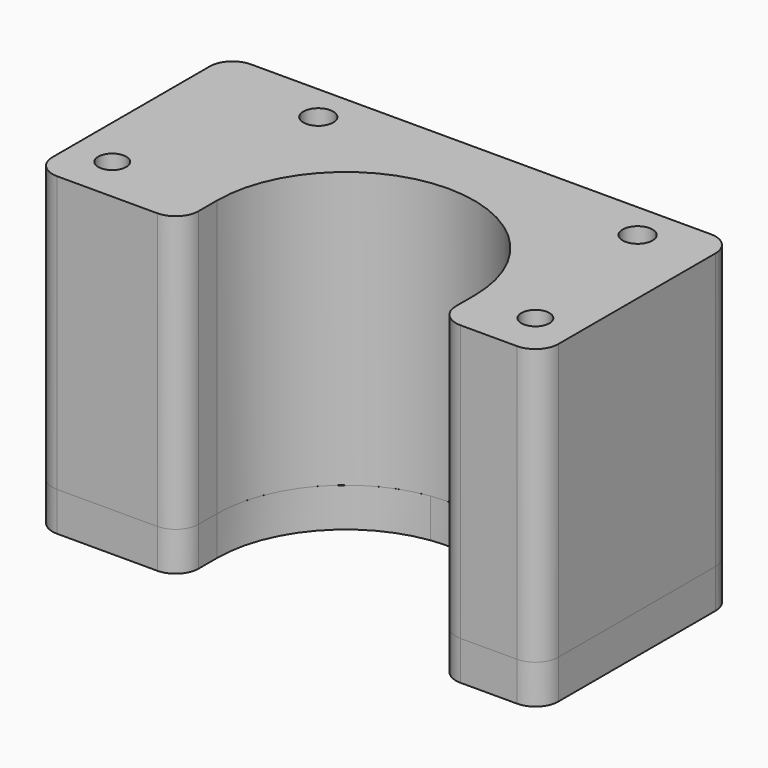
from build123d import *

# Parameters (mm, degrees)
F2_R     = 5.5
F2_R_2   = 3.25
F2_R_3   = 2.5
F2_R_4   = 3.05
F2_R_5   = 2.79
F3_DEPTH = 8.5
F4_R     = 5
F5_R     = 5.5
F5_R_2   = 3.25
F6_DEPTH = 10
F7_R     = 5.5
F7_R_2   = 3.25
F7_R_3   = 3.05
F8_DEPTH = 50


# Not quite as in the source:
# - a feature names something its author has since deleted; it is built from what else it names


with BuildPart() as f3:
    # F2 (on offset) → F3 (new body)
    with BuildSketch(Plane.XY.offset(-60)):
        with BuildLine():
            ThreePointArc((-3.739333985, 27.7491870394), (-12.178842961, 33.2301269514), (-15.455, 42.745))
            Line((-15.455, 42.745), (-59.8, 42.745))
            Line((-59.8, 42.745), (-59.8, -10))
            Line((-59.8, -10), (-28, -10))
            Line((-28, -10), (-28, 0))
            ThreePointArc((-28, 0), (-21.0796270316, 18.429577429), (-3.739333985, 27.7491870394))
        make_face()
        with Locations((-50.8, 0)):
            Circle(F2_R, mode=Mode.SUBTRACT)
        with Locations((-33.75, 34.745)):
            Circle(F2_R_2, mode=Mode.SUBTRACT)
        with BuildLine():
            Line((50.3, 42.745), (15.455, 42.745))
            ThreePointArc((15.455, 42.745), (12.178842961, 33.2301269514), (3.739333985, 27.7491870394))
            ThreePointArc((3.739333985, 27.7491870394), (21.0796270316, 18.429577429), (28, 0))
            Line((28, 0), (28, -10))
            Line((28, -10), (50.3, -10))
            Line((50.3, -10), (50.3, 42.745))
        make_face()
        with Locations((41.3, 0)):
            Circle(F2_R, mode=Mode.SUBTRACT)
        with Locations((35.75, 34.745)):
            Circle(F2_R_2, mode=Mode.SUBTRACT)
        with BuildLine():
            Line((-15.455, 42.745), (15.455, 42.745))
            ThreePointArc((15.455, 42.745), (0, 58.2), (-15.455, 42.745))
        make_face()
        with Locations((0, 52.7)):
            Circle(F2_R_3, mode=Mode.SUBTRACT)
        with BuildLine():
            ThreePointArc((3.739333985, 27.7491870394), (12.178842961, 33.2301269514), (15.455, 42.745))
            Line((15.455, 42.745), (-15.455, 42.745))
            ThreePointArc((-15.455, 42.745), (-12.178842961, 33.2301269514), (-3.739333985, 27.7491870394))
            ThreePointArc((-3.739333985, 27.7491870394), (0, 28), (3.739333985, 27.7491870394))
        make_face()
        with Locations((-50.8, 0)):
            Circle(F2_R)
        with Locations((-50.8, 0)):
            Circle(F2_R_4, mode=Mode.SUBTRACT)
        with Locations((41.3, 0)):
            Circle(F2_R)
        with Locations((41.3, 0)):
            Circle(F2_R_4, mode=Mode.SUBTRACT)
        with Locations((-33.75, 34.745)):
            Circle(F2_R_2)
        with Locations((-33.75, 34.745)):
            Circle(F2_R_5, mode=Mode.SUBTRACT)
        with Locations((35.75, 34.745)):
            Circle(F2_R_2)
        with Locations((35.75, 34.745)):
            Circle(F2_R_5, mode=Mode.SUBTRACT)
    extrude(amount=-F3_DEPTH)

    # F4
    f4_edges = [f3.edges().sort_by_distance(p)[0] for p in [
        (-28, -10, -64.25),
        (28, -10, -64.25),
        (-15.455, 42.745, -64.25),
        (-59.8, 42.745, -64.25),
        (-59.8, -10, -64.25),
        (50.3, -10, -64.25),
        (50.3, 42.745, -64.25),
        (15.455, 42.745, -64.25),
    ]]
    fillet(f4_edges, radius=F4_R)


with BuildPart() as f6:
    # F5 (on face) → F6 (new body)
    with BuildSketch(Plane.XY.offset(-60)):
        with BuildLine():
            ThreePointArc((-28, 0), (0, 28), (28, 0))
            Line((28, 0), (28, -5))
            ThreePointArc((28, -5), (29.4644660941, -8.5355339059), (33, -10))
            Line((33, -10), (45.3, -10))
            ThreePointArc((45.3, -10), (48.8355339059, -8.5355339059), (50.3, -5))
            Line((50.3, -5), (50.3, 37.745))
            ThreePointArc((50.3, 37.745), (48.8355339059, 41.2805339059), (45.3, 42.745))
            Line((45.3, 42.745), (29.041634566, 42.745))
            Line((29.041634566, 42.745), (19.8344907926, 42.745))
            Line((19.8344907926, 42.745), (-19.8344907926, 42.745))
            Line((-19.8344907926, 42.745), (-25.041634566, 42.745))
            Line((-25.041634566, 42.745), (-54.8, 42.745))
            ThreePointArc((-54.8, 42.745), (-58.3355339059, 41.2805339059), (-59.8, 37.745))
            Line((-59.8, 37.745), (-59.8, -5))
            ThreePointArc((-59.8, -5), (-58.3355339059, -8.5355339059), (-54.8, -10))
            Line((-54.8, -10), (-33, -10))
            ThreePointArc((-33, -10), (-29.4644660941, -8.5355339059), (-28, -5))
            Line((-28, -5), (-28, 0))
        make_face()
        with Locations((-50.8, 0)):
            Circle(F5_R, mode=Mode.SUBTRACT)
        with Locations((41.3, 0)):
            Circle(F5_R, mode=Mode.SUBTRACT)
        with Locations((-33.75, 34.745)):
            Circle(F5_R_2, mode=Mode.SUBTRACT)
        with Locations((35.75, 34.745)):
            Circle(F5_R_2, mode=Mode.SUBTRACT)
    extrude(amount=F6_DEPTH)

    # F7 (on face) → F8 (join)
    with BuildSketch(Plane.XY.offset(-50)):
        with BuildLine():
            Line((-28, -5), (-28, 0))
            ThreePointArc((-28, 0), (0, 28), (28, 0))
            Line((28, 0), (28, -5))
            ThreePointArc((28, -5), (29.4644660941, -8.5355339059), (33, -10))
            Line((33, -10), (45.3, -10))
            ThreePointArc((45.3, -10), (48.8355339059, -8.5355339059), (50.3, -5))
            Line((50.3, -5), (50.3, 37.745))
            ThreePointArc((50.3, 37.745), (48.8355339059, 41.2805339059), (45.3, 42.745))
            Line((45.3, 42.745), (-54.8, 42.745))
            ThreePointArc((-54.8, 42.745), (-58.3355339059, 41.2805339059), (-59.8, 37.745))
            Line((-59.8, 37.745), (-59.8, -5))
            ThreePointArc((-59.8, -5), (-58.3355339059, -8.5355339059), (-54.8, -10))
            Line((-54.8, -10), (-33, -10))
            ThreePointArc((-33, -10), (-29.4644660941, -8.5355339059), (-28, -5))
        make_face()
        with Locations((-50.8, 0)):
            Circle(F7_R, mode=Mode.SUBTRACT)
        with Locations((41.3, 0)):
            Circle(F7_R, mode=Mode.SUBTRACT)
        with Locations((-33.75, 34.745)):
            Circle(F7_R_2, mode=Mode.SUBTRACT)
        with Locations((35.75, 34.745)):
            Circle(F7_R_2, mode=Mode.SUBTRACT)
        with Locations((-50.8, 0)):
            Circle(F7_R)
        with Locations((-50.8, 0)):
            Circle(F7_R_3, mode=Mode.SUBTRACT)
        with Locations((41.3, 0)):
            Circle(F7_R)
        with Locations((41.3, 0)):
            Circle(F7_R_3, mode=Mode.SUBTRACT)
    extrude(amount=F8_DEPTH)


solid = Compound([f3.part, f6.part])
